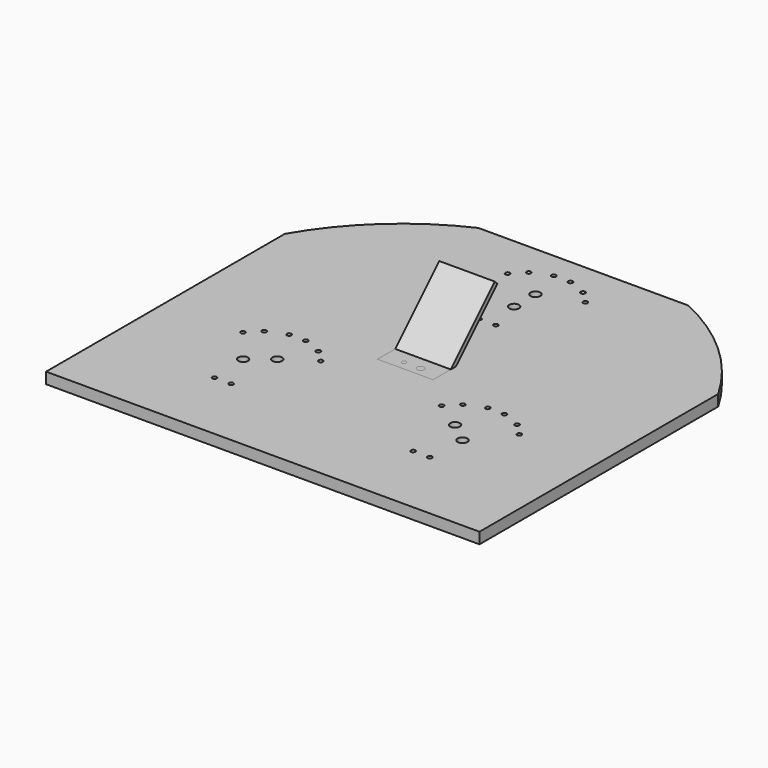
from build123d import *

# Parameters (mm, degrees)
F1_DEPTH  = 10
F2_D      = 8.75
F4_D      = 4.015
F5_D      = 4.038
F7_DEPTH  = 25
F8_R      = 1.9925
F8_R_2    = 3.175
F9_DEPTH  = 4
F10_R     = 4
F11_DEPTH = 1


with BuildPart() as f1:
    # F0 (on Top) → F1 (new body)
    with BuildSketch(Plane.XY):
        with BuildLine():
            Line((-195, -180.25), (195, -180.25))
            Line((195, -180.25), (195, 88.2497216032))
            ThreePointArc((195, 88.2497216032), (151.8246127367, 142.0550720916), (94.3765728346, 180.25))
            Line((94.3765728346, 180.25), (-94.3765728346, 180.25))
            ThreePointArc((-94.3765728346, 180.25), (-151.8246127367, 142.0550720916), (-195, 88.2497216032))
            Line((-195, 88.2497216032), (-195, -180.25))
        make_face()
    extrude(amount=-F1_DEPTH)

    # F2 (through all)
    with Locations(Plane.XY):
        with Locations((0, 126.4499877989), (0, 102.4499877989), (-80, -64), (-98.7408514266, -78.9926811413), (80, -64), (98.7408514266, -78.9926811413)):
            Hole(F2_D / 2)

    # F4 (through all)
    with Locations(Plane.XY):
        with Locations((-7.5, 72.4499877989), (81.8704257133, -113.4963405707), (-96.8704257133, -113.4963405707), (-113.7656096643, -36.4945549019), (-81.8704257133, -29.4963405707), (-54.3686400446, -47.1011566197), (64.9752417624, -36.4945549019), (96.8704257133, -29.4963405707), (124.3722113821, -47.1011566197), (-24.3951839509, 149.4517734677), (7.5, 156.4499877989), (35.0017856687, 138.8451717499)):
            Hole(F4_D / 2)

    # F5 (through all)
    with Locations(Plane.XY):
        with Locations((7.5, 72.4499877989), (24.3951839509, 149.4517734677), (-7.5, 156.4499877989), (-35.0017856687, 138.8451717499), (-81.8704257133, -113.4963405707), (-64.9752417624, -36.4945549019), (-96.8704257133, -29.4963405707), (-124.3722113821, -47.1011566197), (96.8704257133, -113.4963405707), (113.7656096643, -36.4945549019), (81.8704257133, -29.4963405707), (54.3686400446, -47.1011566197)):
            Hole(F5_D / 2)


with BuildPart() as f7:
    # F6 (on Right) → F7 (new body, symmetric)
    with BuildSketch(Plane.YZ):
        with BuildLine():
            Line((49.4974746831, 49.4974746831), (0, 0))
            Line((0, 0), (-20, 0))
            Line((-20, 0), (-20, -4))
            Line((-20, -4), (0, -4))
            ThreePointArc((0, -4), (1.5307337295, -3.69551813), (2.8284271247, -2.8284271247))
            Line((2.8284271247, -2.8284271247), (52.3259018078, 46.6690475583))
            Line((52.3259018078, 46.6690475583), (49.4974746831, 49.4974746831))
        make_face()
    extrude(amount=F7_DEPTH, both=True)

    # F8 (on face) → F9 (cut, through all)
    with BuildSketch(Plane.XY):
        with Locations((-7.5, -12)):
            Circle(F8_R)
        with Locations((7.5, -12)):
            Circle(F8_R_2)
    extrude(amount=-F9_DEPTH, mode=Mode.SUBTRACT)

    # F10 (on face) → F11 (cut)
    with BuildSketch(Plane(origin=(0, 0, -4), x_dir=(1, 0, 0), z_dir=(0, 0, -1))):
        with Locations((7.5, 12)):
            Circle(F10_R)
    extrude(amount=-F11_DEPTH, mode=Mode.SUBTRACT)


solid = Compound([f1.part, f7.part])
